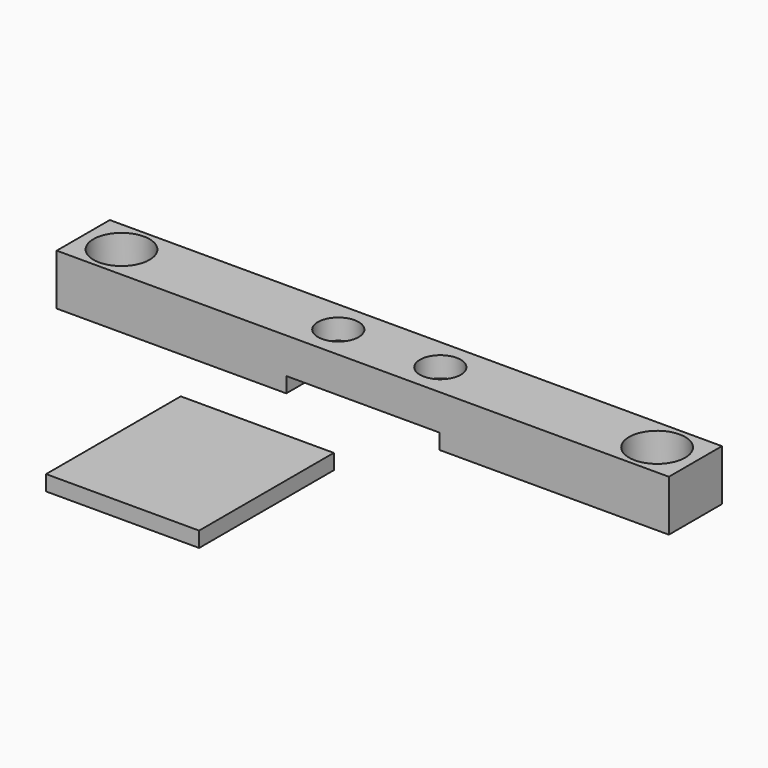
from build123d import *

# Parameters (mm, degrees)
F0_W     = 120
F0_H     = 13
F0_R     = 5.5
F0_R_2   = 4
F0_R_3   = 1.65
F1_DEPTH = 10
F2_DEPTH = 7
F4_DEPTH = 25
F5_DEPTH = 4
F0_W_2   = 30
F0_H_2   = 33
F6_DEPTH = 3


# Not quite as in the source:
# - a feature names something its author has since deleted; it is built from what else it names


with BuildPart() as f1:
    # F0 (on Top) → F1 (new body)
    with BuildSketch(Plane.XY):
        Rectangle(F0_W, F0_H)
        with Locations((-52.5, 0)):
            Circle(F0_R, mode=Mode.SUBTRACT)
        with Locations((-10, 0)):
            Circle(F0_R_2, mode=Mode.SUBTRACT)
        with Locations((10, 0)):
            Circle(F0_R_2, mode=Mode.SUBTRACT)
        with Locations((52.5, 0)):
            Circle(F0_R, mode=Mode.SUBTRACT)
        with Locations((-52.5, 0)):
            Circle(F0_R)
        with BuildLine():
            ThreePointArc((-55.5, 0), (-54.6213203436, 2.1213203436), (-52.5, 3))
            ThreePointArc((-52.5, 3), (-50.3786796564, 2.1213203436), (-49.5, 0))
            ThreePointArc((-49.5, 0), (-50.3786796564, -2.1213203436), (-52.5, -3))
            ThreePointArc((-52.5, -3), (-54.6213203436, -2.1213203436), (-55.5, 0))
        make_face(mode=Mode.SUBTRACT)
        with Locations((52.5, 0)):
            Circle(F0_R)
        with BuildLine():
            ThreePointArc((52.5, 3), (54.6213203436, 2.1213203436), (55.5, 0))
            ThreePointArc((55.5, 0), (54.6213203436, -2.1213203436), (52.5, -3))
            ThreePointArc((52.5, -3), (50.3786796564, -2.1213203436), (49.5, 0))
            ThreePointArc((49.5, 0), (50.3786796564, 2.1213203436), (52.5, 3))
        make_face(mode=Mode.SUBTRACT)
        with Locations((-10, 0)):
            Circle(F0_R_2)
        with Locations((-10, 0)):
            Circle(F0_R_3, mode=Mode.SUBTRACT)
        with Locations((10, 0)):
            Circle(F0_R_2)
        with Locations((10, 0)):
            Circle(F0_R_3, mode=Mode.SUBTRACT)
    extrude(amount=-F1_DEPTH)

    # F0 (on Top) → F2 (cut)
    with BuildSketch(Plane.XY):
        with Locations((-52.5, 0)):
            Circle(F0_R)
        with BuildLine():
            ThreePointArc((-55.5, 0), (-54.6213203436, 2.1213203436), (-52.5, 3))
            ThreePointArc((-52.5, 3), (-50.3786796564, 2.1213203436), (-49.5, 0))
            ThreePointArc((-49.5, 0), (-50.3786796564, -2.1213203436), (-52.5, -3))
            ThreePointArc((-52.5, -3), (-54.6213203436, -2.1213203436), (-55.5, 0))
        make_face(mode=Mode.SUBTRACT)
        with Locations((52.5, 0)):
            Circle(F0_R)
        with BuildLine():
            ThreePointArc((52.5, 3), (54.6213203436, 2.1213203436), (55.5, 0))
            ThreePointArc((55.5, 0), (54.6213203436, -2.1213203436), (52.5, -3))
            ThreePointArc((52.5, -3), (50.3786796564, -2.1213203436), (49.5, 0))
            ThreePointArc((49.5, 0), (50.3786796564, 2.1213203436), (52.5, 3))
        make_face(mode=Mode.SUBTRACT)
    extrude(amount=-F2_DEPTH, mode=Mode.SUBTRACT)

    # F3 (on face) → F4 (cut)
    with BuildSketch(Plane.XZ.offset(6.5)):
        Polygon((-15, -10), (0, -10), (15, -10), (15, -7), (0, -7), (-15, -7), align=None)
    extrude(amount=-F4_DEPTH, mode=Mode.SUBTRACT)

    # F0 (on Top) → F5 (cut)
    with BuildSketch(Plane.XY):
        with Locations((-10, 0)):
            Circle(F0_R_2)
        with Locations((-10, 0)):
            Circle(F0_R_3, mode=Mode.SUBTRACT)
        with Locations((10, 0)):
            Circle(F0_R_2)
        with Locations((10, 0)):
            Circle(F0_R_3, mode=Mode.SUBTRACT)
    extrude(amount=-F5_DEPTH, mode=Mode.SUBTRACT)


with BuildPart() as f6:
    # F0 (on Top) → F6 (new body)
    with BuildSketch(Plane.XY):
        with Locations((0, -48.8559566438)):
            Rectangle(F0_W_2, F0_H_2)
    extrude(amount=-F6_DEPTH)


solid = Compound([f1.part, f6.part])
